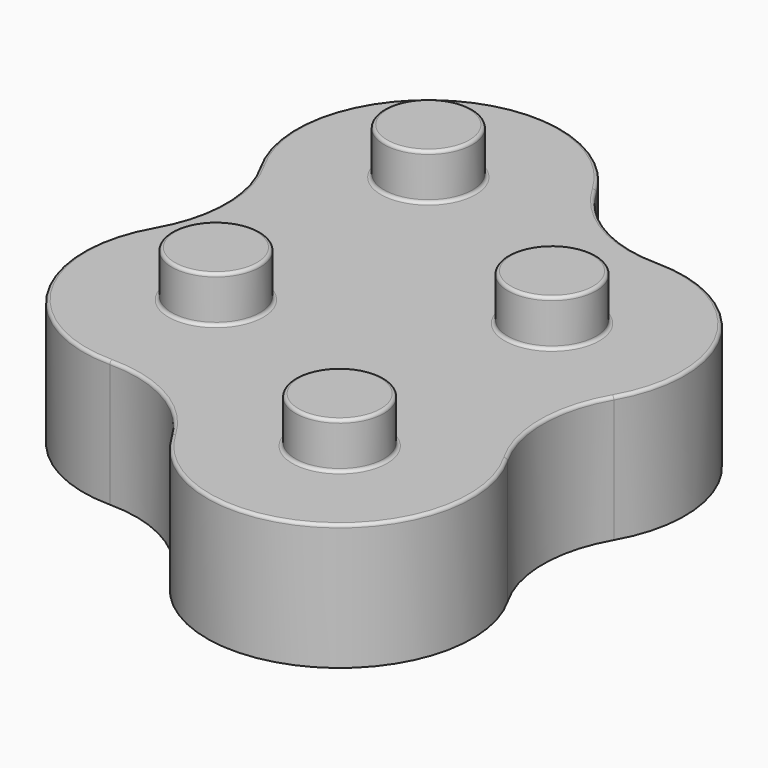
from build123d import *

# Parameters (mm, degrees)
F4_R     = 7.9
F5_DEPTH = 20
F6_DEPTH = 10
F7_R     = 7
F8_DEPTH = 7.3
F9_R     = 0.5


# Not quite as in the source:
# - a feature names something its author has since deleted; it is built from what else it names


with BuildPart() as f5:
    # F4 (on Top) → F5 (new body)
    with BuildSketch(Plane.XY):
        with BuildLine():
            ThreePointArc((18.1865334795, 10.5), (15.3730669589, 21), (18.1865334795, 31.5))
            ThreePointArc((18.1865334795, 31.5), (18.1865334795, 52.5), (0, 63))
            ThreePointArc((0, 63), (-10.5, 65.8134665205), (-18.1865334795, 73.5))
            ThreePointArc((-18.1865334795, 73.5), (-46.8730669589, 81.1865334795), (-54.5596004384, 52.5))
            ThreePointArc((-54.5596004384, 52.5), (-51.7461339179, 42), (-54.5596004384, 31.5))
            ThreePointArc((-54.5596004384, 31.5), (-54.5596004384, 10.5), (-36.3730669589, 0))
            ThreePointArc((-36.3730669589, 0), (-25.8730669589, -2.8134665205), (-18.1865334795, -10.5))
            ThreePointArc((-18.1865334795, -10.5), (10.5, -18.1865334795), (18.1865334795, 10.5))
        make_face()
        with Locations((-36.3730669589, 21)):
            Circle(F4_R, mode=Mode.SUBTRACT)
        Circle(F4_R, mode=Mode.SUBTRACT)
        with Locations((-36.3730669589, 63)):
            Circle(F4_R, mode=Mode.SUBTRACT)
        with Locations((0, 42)):
            Circle(F4_R, mode=Mode.SUBTRACT)
        with Locations((0, 42)):
            Circle(F4_R)
        Circle(F4_R)
        with Locations((-36.3730669589, 21)):
            Circle(F4_R)
        with Locations((-36.3730669589, 63)):
            Circle(F4_R)
    extrude(amount=F5_DEPTH)

    # F4 (on Top) → F6 (cut)
    with BuildSketch(Plane.XY):
        with Locations((0, 42)):
            Circle(F4_R)
        Circle(F4_R)
        with Locations((-36.3730669589, 21)):
            Circle(F4_R)
        with Locations((-36.3730669589, 63)):
            Circle(F4_R)
    extrude(amount=F6_DEPTH, mode=Mode.SUBTRACT)

    # F7 (on face) → F8 (join)
    with BuildSketch(Plane.XY.offset(20)):
        Circle(F7_R)
        with Locations((0, 42)):
            Circle(F7_R)
        with Locations((-36.3730669589, 21)):
            Circle(F7_R)
        with Locations((-36.3730669589, 63)):
            Circle(F7_R)
    extrude(amount=F8_DEPTH)

    # F9
    f9_edges = [f5.edges().sort_by_distance(p)[0] for p in [
        (-7, 0, 27.3),
        (-7.9, 42, 0),
        (-7.9, 42, 10),
        (-7.9, 0, 0),
        (-7.9, 0, 10),
        (-7, 42, 27.3),
        (-7, 42, 20),
        (18.186533, 52.5, 20),
        (-43.373067, 21, 20),
        (-43.373067, 21, 27.3),
        (-28.473067, 21, 5),
        (-44.273067, 21, 0),
        (-44.273067, 21, 10),
        (-29.373067, 63, 23.65),
        (-43.373067, 63, 20),
        (-43.373067, 63, 27.3),
        (-28.473067, 63, 5),
        (-44.273067, 63, 0),
        (-44.273067, 63, 10),
        (7, 0, 23.65),
        (-7, 0, 20),
    ]]
    fillet(f9_edges, radius=F9_R)


solid = f5.part
